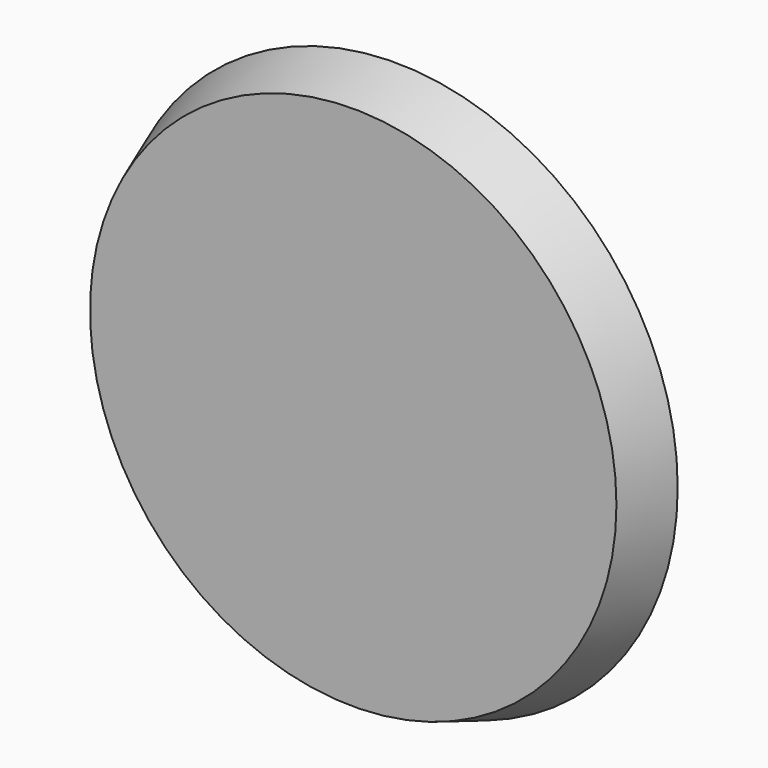
from build123d import *

# Parameters (mm, degrees)
F0_R     = 300
F1_DEPTH = 50


# Not quite as in the source:
# - a fillet or chamfer that OpenCascade refuses, or shapes differently, is made with other operations: its cross-section is extruded or revolved along the edge and cut away or added


with BuildPart() as f1:
    # F0 (on Front) → F1 (new body)
    with BuildSketch(Plane.XZ):
        Circle(F0_R)
    extrude(amount=F1_DEPTH)

    # F2: chamfer of 50 x 137.3738709727 on 1 edges, made by hand

    # F2_s1 → F2_t2 (revolve, cut)
    with BuildSketch(Plane.XY):
        Polygon((300, 87.3738709727), (250, -50), (300, -50), align=None)
    revolve(axis=Axis((0, -50, 0), (0, -1, 0)), mode=Mode.SUBTRACT)


solid = f1.part
